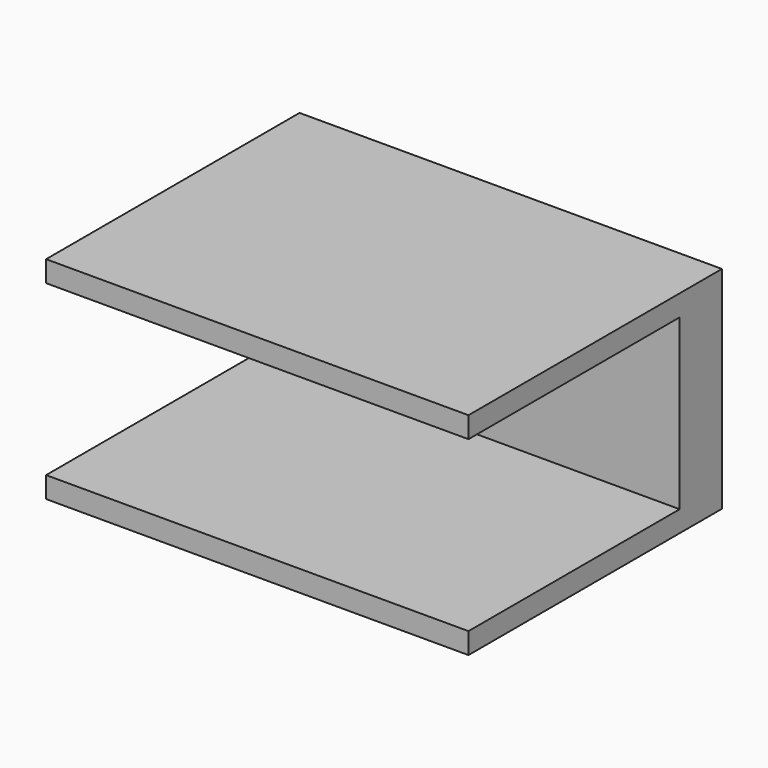
from build123d import *

# Parameters (mm, degrees)
F0_W     = 101.6
F0_H     = 50.8
F1_DEPTH = 76.2
F3_W     = 101.6
F3_H     = 40.64
F4_DEPTH = 63.5


# Not quite as in the source:
# - the program builds the solid bodies; features that only make, move or delete a surface that nothing else refers to are left out


with BuildPart() as f1:
    # F0 (on Front) → F1 (new body)
    with BuildSketch(Plane.XZ):
        with Locations((0.3947839141, -13.1712006897)):
            Rectangle(F0_W, F0_H)
    extrude(amount=-F1_DEPTH)

    # F3 (on face) → F4 (cut)
    with BuildSketch(Plane.XZ):
        with Locations((0.3947839141, -13.1712006897)):
            Rectangle(F3_W, F3_H)
    extrude(amount=-F4_DEPTH, mode=Mode.SUBTRACT)


solid = f1.part
